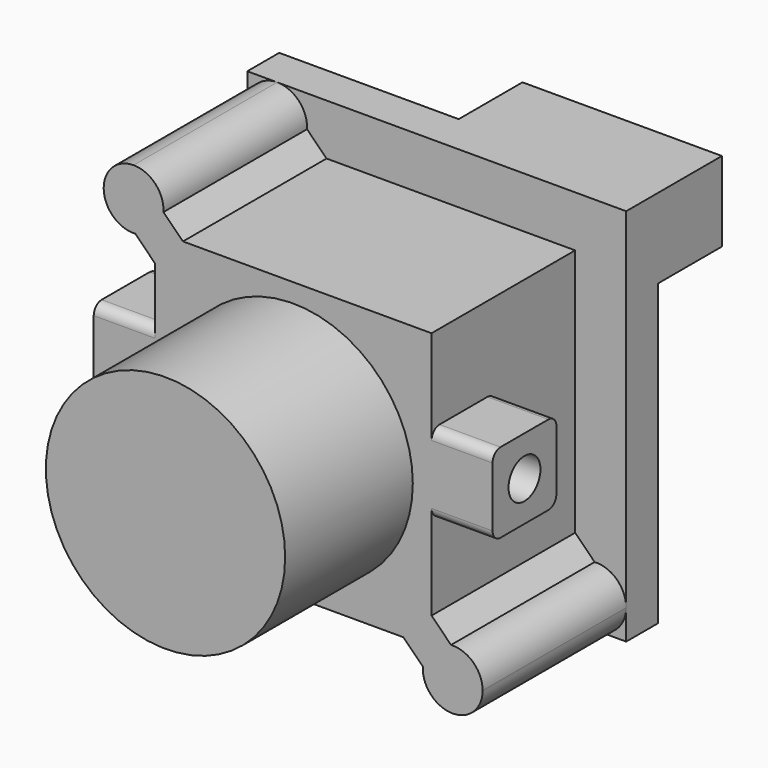
from build123d import *

# Parameters (mm, degrees)
F0_W      = 19
F0_H      = 19
F1_DEPTH  = 2
F4_DEPTH  = 9
F2_R      = 6
F5_DEPTH  = 17
F7_DEPTH  = 10
F10_R     = 1
F11_DEPTH = 20
F12_W     = 10
F12_H     = 4
F13_DEPTH = 4


# Not quite as in the source:
# - a feature of the source that left no trace in its solid (it failed there, or was rolled back) is left out
# - a feature names something its author has since deleted; it is built from what else it names


with BuildPart() as f1:
    # F0 (on Front) → F1 (new body)
    with BuildSketch(Plane.XZ):
        Rectangle(F0_W, F0_H)
    extrude(amount=F1_DEPTH)

    # F3 (on face) → F4 (join)
    with BuildSketch(Plane.XZ.offset(2)):
        with BuildLine():
            Line((-5.5251262658, 6.9393398282), (-6.5023238038, 7.9165373661))
            ThreePointArc((-6.5023238038, 7.9165373661), (-6.9102307697, 9.0307293654), (-8, 9.5))
            ThreePointArc((-8, 9.5), (-9.0606601718, 9.0606601718), (-9.5, 8))
            ThreePointArc((-9.5, 8), (-9.0307293654, 6.9102307697), (-7.9165373661, 6.5023238038))
            Line((-7.9165373661, 6.5023238038), (-6.9393398282, 5.5251262658))
            Line((-6.9393398282, 5.5251262658), (-6.9393398282, -6.9393398282))
            Line((-6.9393398282, -6.9393398282), (5.5251262658, -6.9393398282))
            Line((5.5251262658, -6.9393398282), (6.5023238038, -7.9165373661))
            ThreePointArc((6.5023238038, -7.9165373661), (6.9102307697, -9.0307293654), (8, -9.5))
            ThreePointArc((8, -9.5), (9.0606601718, -9.0606601718), (9.5, -8))
            ThreePointArc((9.5, -8), (9.0307293654, -6.9102307697), (7.9165373661, -6.5023238038))
            Line((7.9165373661, -6.5023238038), (6.9393398282, -5.5251262658))
            Line((6.9393398282, -5.5251262658), (6.9393398282, 6.9393398282))
            Line((6.9393398282, 6.9393398282), (-5.5251262658, 6.9393398282))
        make_face()
    extrude(amount=F4_DEPTH)

    # F2 (on face) → F5 (join)
    with BuildSketch(Plane.XZ.offset(2)):
        Circle(F2_R)
    extrude(amount=F5_DEPTH)

    # F6 (on Right) → F7 (join, symmetric)
    with BuildSketch(Plane.YZ):
        with BuildLine():
            ThreePointArc((-7, 2.2071067812), (-7.1464466094, 2.5606601718), (-7.5, 2.7071067812))
            Line((-7.5, 2.7071067812), (-10.5, 2.7071067812))
            ThreePointArc((-10.5, 2.7071067812), (-10.8535533906, 2.5606601718), (-11, 2.2071067812))
            Line((-11, 2.2071067812), (-11, -0.7928932188))
            ThreePointArc((-11, -0.7928932188), (-10.8535533906, -1.1464466094), (-10.5, -1.2928932188))
            Line((-10.5, -1.2928932188), (-7.5, -1.2928932188))
            ThreePointArc((-7.5, -1.2928932188), (-7.1464466094, -1.1464466094), (-7, -0.7928932188))
            Line((-7, -0.7928932188), (-7, 2.2071067812))
        make_face()
    extrude(amount=F7_DEPTH, both=True)

    # F10 (on face) → F11 (cut, symmetric)
    with BuildSketch(Plane.YZ.offset(6.9393398282)):
        with Locations((-9, 0.7071067812)):
            Circle(F10_R)
    extrude(amount=F11_DEPTH, both=True, mode=Mode.SUBTRACT)

    # F12 (on face) → F13 (join)
    with BuildSketch(Plane(origin=(0, 0, 0), x_dir=(-1, 0, 0), z_dir=(0, 1, 0))):
        with Locations((-4.5, 7.5)):
            Rectangle(F12_W, F12_H)
    extrude(amount=F13_DEPTH)


solid = f1.part
